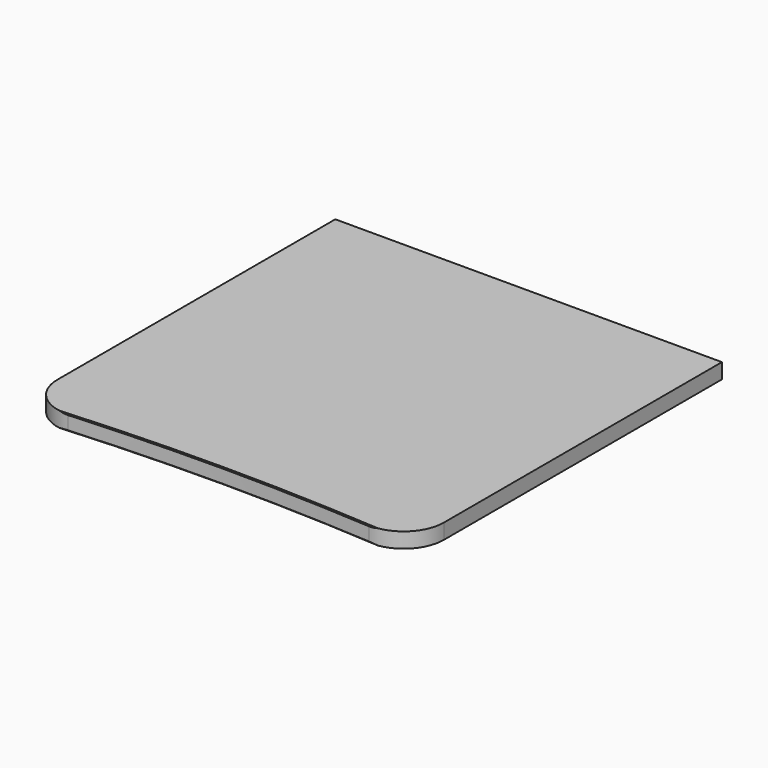
from build123d import *

# Parameters (mm, degrees)
F1_DEPTH    = 12
F2_T2_ANGLE = 8.0362657393
F2_T4_ANGLE = 8.0362657393


# Not quite as in the source:
# - a fillet or chamfer that OpenCascade refuses, or shapes differently, is made with other operations: its cross-section is extruded or revolved along the edge and cut away or added


with BuildPart() as f1:
    # F0 (on Top) → F1 (new body)
    with BuildSketch(Plane.XY):
        with BuildLine():
            Line((152.4, 150.8755259808), (-152.4, 150.8755259808))
            Line((-152.4, 150.8755259808), (-152.4, -123.0348219055))
            ThreePointArc((-152.4, -123.0348219055), (-142.3618011799, -146.2007492455), (-118.5946337308, -154.7182240192))
            ThreePointArc((-118.5946337308, -154.7182240192), (0, -150.8755259808), (118.5946337308, -154.7182240192))
            ThreePointArc((118.5946337308, -154.7182240192), (142.3618011799, -146.2007492455), (152.4, -123.0348219055))
            Line((152.4, -123.0348219055), (152.4, 150.8755259808))
        make_face()
    extrude(amount=F1_DEPTH)

    # F2: chamfer of 0.762 on 2 edges, made by hand

    # F2_s1 → F2_t2 (revolve, cut)
    with BuildSketch(Plane(origin=(-138.6011225893, -9.7360143416, 0), x_dir=(0, 0, 1), z_dir=(-0.9975419239, -0.0700721776, 0))):
        Polygon((11.238, -146.0015284816), (12, -145.2395284816), (12, -146.0015284816), align=None)
    revolve(axis=Axis((0, -1982.8505259812, 12), (0, 0, -1)), revolution_arc=F2_T2_ANGLE, mode=Mode.SUBTRACT)

    # F2_s3 → F2_t4 (revolve, cut)
    with BuildSketch(Plane(origin=(-138.6011225893, -9.7360143416, 0), x_dir=(0, 0, 1), z_dir=(-0.9975419239, -0.0700721776, 0))):
        Polygon((0.762, -146.0015284816), (0, -145.2395284816), (0, -146.0015284816), align=None)
    revolve(axis=Axis((0, -1982.8505259812, 0), (0, 0, -1)), revolution_arc=F2_T4_ANGLE, mode=Mode.SUBTRACT)


solid = f1.part
